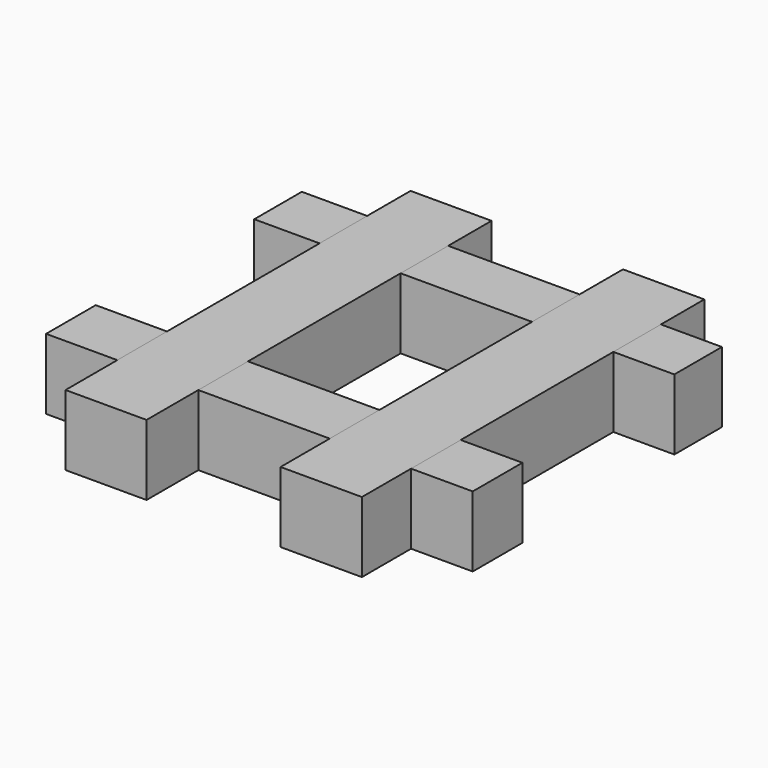
from build123d import *

# Parameters (mm, degrees)
F1_W     = 151.3130292296
F1_H     = 21.4144438505
F2_DEPTH = 25.4
F3_W     = 153.6662653089
F3_H     = 22.3557390273
F4_DEPTH = 25.4
F5_W     = 29.1801150888
F5_H     = 155.3135290742
F6_DEPTH = 25.4
F7_W     = 29.2942132801
F7_H     = 154.1548073292
F8_DEPTH = 25.4


# Not quite as in the source:
# - a feature of the source that left no trace in its solid (it failed there, or was rolled back) is left out


with BuildPart() as f2:
    # F1 (on Top) → F2 (new body)
    with BuildSketch(Plane.XY):
        with Locations((0.7059685886, 45.7704290748)):
            Rectangle(F1_W, F1_H)
    extrude(amount=F2_DEPTH)


with BuildPart() as f4:
    # F3 (on Top) → F4 (new body)
    with BuildSketch(Plane.XY):
        with Locations((-0.2353228629, -44.8291320354)):
            Rectangle(F3_W, F3_H)
    extrude(amount=F4_DEPTH)


with BuildPart() as f6:
    # F5 (on Top) → F6 (new body)
    with BuildSketch(Plane.XY):
        with Locations((-36.8281314149, -1.6472674906)):
            Rectangle(F5_W, F5_H)
    extrude(amount=F6_DEPTH)


with BuildPart() as f8:
    # F7 (on Top) → F8 (new body)
    with BuildSketch(Plane.XY):
        with Locations((39.744076319, -1.07178092)):
            Rectangle(F7_W, F7_H)
    extrude(amount=F8_DEPTH)


solid = Compound([f2.part, f4.part, f6.part, f8.part])
